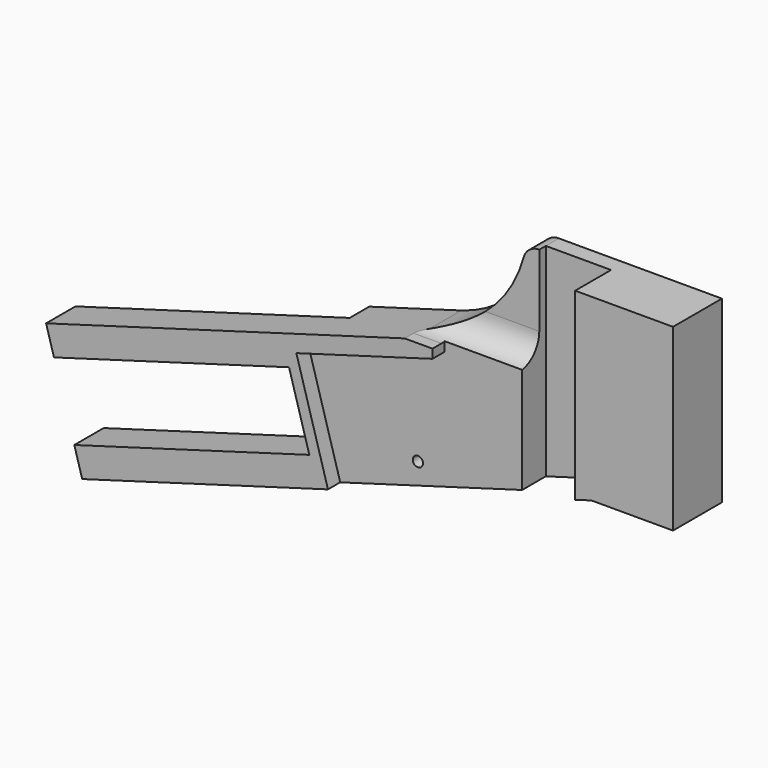
from build123d import *

# Parameters (mm, degrees)
F1_DEPTH  = 19.05
F3_DEPTH  = 13.97
F5_DEPTH  = 7.62
F7_DEPTH  = 11.43
F8_R      = 7.9375
F9_R      = 1.5875
F10_DEPTH = 4.7625
F11_DEPTH = 19.0510001


# Not quite as in the source:
# - a feature names something its author has since deleted; it is built from what else it names


with BuildPart() as f1:
    # F0 (on Front) → F1 (new body)
    with BuildSketch(Plane.XZ):
        Polygon((0, -55.88), (0, 0), (-30.48, 0), (-30.48, -57.344024155), (-25.4, -55.88), align=None)
        with BuildLine():
            Line((-50.8, -63.2001207751), (-50.8, 0))
            ThreePointArc((-50.8, 0), (-53.8879738976, -1.0462898954), (-55.7039336667, -3.7541664537))
            ThreePointArc((-55.7039336667, -3.7541664537), (-65.0479350522, -20.0515789601), (-81.1885565746, -29.6638811382))
            Line((-81.1885565746, -29.6638811382), (-195.2974379776, -62.5493454446))
            Line((-195.2974379776, -62.5493454446), (-192.8355918237, -71.0916761286))
            Line((-192.8355918237, -71.0916761286), (-119.6156145323, -49.990137667))
            Line((-119.6156145323, -49.990137667), (-113.2851529938, -71.9561308545))
            Line((-113.2851529938, -71.9561308545), (-186.5051302853, -93.057669316))
            Line((-186.5051302853, -93.057669316), (-184.0432841314, -101.6))
            Line((-184.0432841314, -101.6), (-50.8, -63.2001207751))
        make_face()
        Polygon((-30.48, -57.344024155), (-30.48, 0), (-50.8, 0), (-50.8, -63.2001207751), align=None)
    extrude(amount=F1_DEPTH)

    # F2 (on face) → F3 (cut)
    with BuildSketch(Plane.XZ.offset(19.05)):
        Polygon((-30.48, 0), (-50.8, 0), (-50.8, -63.2001207751), (-30.48, -57.344024155), align=None)
    extrude(amount=-F3_DEPTH, mode=Mode.SUBTRACT)

    # F4 (on face) → F5 (cut)
    with BuildSketch(Plane.XZ):
        Polygon((-109.8741311376, -37.9308839061), (-195.2974379776, -62.5493454446), (-184.0432841314, -101.6), (-98.6199772914, -76.9815384615), align=None)
    extrude(amount=F5_DEPTH, mode=Mode.SUBTRACT)

    # F6 (on face) → F7 (cut)
    with BuildSketch(Plane.XZ.offset(19.05)):
        with BuildLine():
            Line((-83.9840349336, -30.353), (-50.8, -30.353))
            Line((-50.8, -30.353), (-50.8, 0))
            ThreePointArc((-50.8, 0), (-53.8879738976, -1.0462898954), (-55.7039336667, -3.7541664537))
            ThreePointArc((-55.7039336667, -3.7541664537), (-66.0773822208, -21.0582659153), (-83.9840349336, -30.353))
        make_face()
    extrude(amount=-F7_DEPTH, mode=Mode.SUBTRACT)

    # F8
    f8_edges = [f1.edges().sort_by_distance(p)[0] for p in [
        (-67.189861, -7.62, -30.353),
    ]]
    fillet(f8_edges, radius=F8_R)

    # F9 (on face) → F10 (cut)
    with BuildSketch(Plane.XZ.offset(19.05)):
        with BuildLine():
            Line((-78.4844835363, -71.1786153846), (-73.6695687, -69.790987112))
            ThreePointArc((-73.6695687, -69.7909871121), (-78.2220260856, -57.0610953752), (-78.0424581585, -43.5428570566))
            ThreePointArc((-78.0424581585, -43.5428570566), (-76.567170767, -38.1173977165), (-74.3094881962, -32.9681306475))
            Line((-74.3094881962, -32.9681306475), (-74.93, -33.1469582596))
            Line((-74.93, -33.1469582596), (-84.154369829, -35.8053638195))
            Line((-84.154369829, -35.8053638195), (-117.3289133872, -45.3660593118))
            Line((-117.3289133872, -45.3660593118), (-107.4815287718, -79.5353820478))
            Line((-107.4815287718, -79.5353820478), (-94.3488119494, -75.7506153846))
            Line((-94.3488119494, -75.7506153846), (-96.9865042571, -66.5981182232))
            Line((-96.9865042571, -66.5981182232), (-81.122175844, -62.0261182232))
            Line((-81.122175844, -62.0261182232), (-78.4844835363, -71.1786153846))
        make_face()
        Polygon((-86.4166477429, -73.4646153846), (-78.4844835363, -71.1786153846), (-81.122175844, -62.0261182232), (-96.9865042571, -66.5981182232), (-94.3488119494, -75.7506153846), align=None)
        with Locations((-93.0564411007, -68.7697198411)):
            Circle(F9_R, mode=Mode.SUBTRACT)
        with Locations((-83.2937774619, -65.9561813796)):
            Circle(F9_R, mode=Mode.SUBTRACT)
        with Locations((-83.2937774619, -65.9561813796)):
            Circle(F9_R)
        with Locations((-93.0564411007, -68.7697198411)):
            Circle(F9_R)
        with BuildLine():
            ThreePointArc((-78.0424581585, -43.5428570566), (-78.2220260856, -57.0610953752), (-73.6695687, -69.7909871121))
            Line((-73.6695687, -69.790987112), (-50.8, -63.2001207751))
            Line((-50.8, -63.2001207751), (-50.8, -53.6799892795))
            Line((-50.8, -53.6799892795), (-74.2742938603, -49.1253072525))
            ThreePointArc((-74.2742938603, -49.1253072525), (-77.3145392982, -47.1144945318), (-78.0424581585, -43.5428570566))
        make_face()
        with BuildLine():
            ThreePointArc((-74.3094881962, -32.9681306475), (-76.567170767, -38.1173977165), (-78.0424581585, -43.5428570566))
            ThreePointArc((-78.0424581585, -43.5428570566), (-72.9114890511, -39.7093483015), (-68.6046509033, -44.45))
            ThreePointArc((-68.6046509033, -44.45), (-70.3372055311, -48.1243485533), (-74.2742938603, -49.1253072525))
            Line((-74.2742938603, -49.1253072525), (-50.8, -53.6799892795))
            Line((-50.8, -53.6799892795), (-50.8, -42.2880161767))
            ThreePointArc((-50.8, -42.2880161767), (-54.8534085622, -36.9235653105), (-56.279986835, -30.353))
            Line((-56.279986835, -30.353), (-65.2352774711, -30.353))
            Line((-65.2352774711, -30.353), (-74.3094881962, -32.9681306475))
        make_face()
        with BuildLine():
            ThreePointArc((-68.6046509033, -44.45), (-72.9114890511, -39.7093483015), (-78.0424581585, -43.5428570566))
            ThreePointArc((-78.0424581585, -43.5428570566), (-77.3145392982, -47.1144945318), (-74.2742938603, -49.1253072525))
            ThreePointArc((-74.2742938603, -49.1253072525), (-70.3372055311, -48.1243485533), (-68.6046509033, -44.45))
        make_face()
        with BuildLine():
            Line((-50.8, -30.353), (-56.279986835, -30.353))
            ThreePointArc((-56.279986835, -30.353), (-54.8534085622, -36.9235653105), (-50.8, -42.2880161767))
            Line((-50.8, -42.2880161767), (-50.8, -30.353))
        make_face()
        with BuildLine():
            Line((-50.8, -28.4059811383), (-56.1527436573, -28.4059811383))
            ThreePointArc((-56.1527436573, -28.4059811383), (-56.2467573472, -29.3775043596), (-56.279986835, -30.353))
            Line((-56.279986835, -30.353), (-50.8, -30.353))
            Line((-50.8, -30.353), (-50.8, -28.4059811383))
        make_face()
        with BuildLine():
            Line((-56.1527436573, -28.4059811383), (-71.4639828579, -28.4059811383))
            ThreePointArc((-71.4639828579, -28.4059811383), (-72.1413197609, -29.3692544852), (-72.7885643692, -30.353))
            Line((-72.7885643692, -30.353), (-65.2352774711, -30.353))
            Line((-65.2352774711, -30.353), (-56.279986835, -30.353))
            ThreePointArc((-56.279986835, -30.353), (-56.2467573472, -29.3775043596), (-56.1527436573, -28.4059811383))
        make_face()
        with BuildLine():
            ThreePointArc((-72.7885643692, -30.353), (-72.1413197609, -29.3692544852), (-71.4639828579, -28.4059811383))
            Line((-71.4639828579, -28.4059811383), (-74.93, -28.4059811383))
            Line((-74.93, -28.4059811383), (-74.93, -30.353))
            Line((-74.93, -30.353), (-72.7885643692, -30.353))
        make_face()
        with BuildLine():
            ThreePointArc((-72.7885643692, -30.353), (-73.5749926059, -31.6454636692), (-74.3094881962, -32.9681306475))
            Line((-74.3094881962, -32.9681306475), (-65.2352774711, -30.353))
            Line((-65.2352774711, -30.353), (-72.7885643692, -30.353))
        make_face()
        with BuildLine():
            Line((-74.93, -33.1469582596), (-74.3094881962, -32.9681306475))
            ThreePointArc((-74.3094881962, -32.9681306475), (-73.5749926059, -31.6454636692), (-72.7885643692, -30.353))
            Line((-72.7885643692, -30.353), (-74.93, -30.353))
            Line((-74.93, -30.353), (-74.93, -33.1469582596))
        make_face()
    extrude(amount=-F10_DEPTH, mode=Mode.SUBTRACT)

    # F9 (on face) → F11 (cut, through all)
    with BuildSketch(Plane.XZ.offset(19.05)):
        with Locations((-83.2937774619, -65.9561813796)):
            Circle(F9_R)
    extrude(amount=-F11_DEPTH, mode=Mode.SUBTRACT)


solid = f1.part
